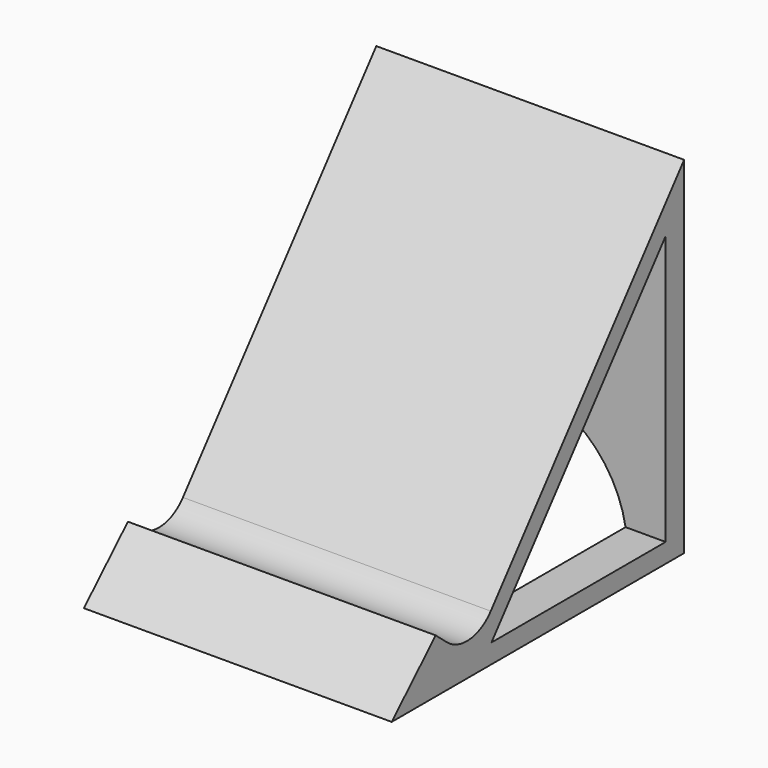
from build123d import *

# Parameters (mm, degrees)
F1_DEPTH = 101.6
F3_REACH = 205.8451899427


with BuildPart() as f1:
    # F0 (on Right) → F1 (new body)
    with BuildSketch(Plane.YZ):
        with BuildLine():
            Line((-36.1766421175, -23.2471508509), (-54.3283293044, -41.0144312356))
            Line((-54.3283293044, -41.0144312356), (58.7016706956, -41.0144312356))
            Line((58.7016706956, -41.0144312356), (58.7016706956, -34.6644312356))
            Line((58.7016706956, -34.6644312356), (-13.140378273, -34.6644312356))
            Line((-13.140378273, -34.6644312356), (58.7016706956, 54.2355687644))
            Line((58.7016706956, 54.2355687644), (66.3216706956, 54.2355687644))
            Line((66.3216706956, 54.2355687644), (66.3216706956, 73.2855687644))
            Line((66.3216706956, 73.2855687644), (-13.4575252541, -25.4361495295))
            ThreePointArc((-13.4575252541, -25.4361495295), (-22.1196896865, -30.0953879884), (-31.5109779006, -27.1721532474))
            Line((-31.5109779006, -27.1721532474), (-36.1766421175, -23.2471508509))
        make_face()
        Polygon((58.7016706956, -34.6644312356), (58.7016706956, -41.0144312356), (66.3216706956, -41.0144312356), (66.3216706956, 54.2355687644), (58.7016706956, 54.2355687644), align=None)
    extrude(amount=F1_DEPTH)

    f3_end = Plane(origin=(50.8, 22.7806462113, 9.7855687644), x_dir=(0, 0.6285393611, 0.7777777778), z_dir=(0, 0.7777777778, -0.6285393611))
    # F2 (on face) → F3 (cut, up to a plane its end follows)
    with BuildSketch(Plane(origin=(0, 66.3216706956, 0), x_dir=(-1, 0, 0), z_dir=(0, 1, 0))):
        with BuildLine():
            Line((-88.9, -41.0144312356), (-12.7, -41.0144312356))
            ThreePointArc((-12.7, -41.0144312356), (-50.8, -2.9144312356), (-88.9, -41.0144312356))
        make_face()
    f3_long = extrude(amount=-F3_REACH, mode=Mode.PRIVATE)
    add(split(f3_long, bisect_by=f3_end, keep=Keep.TOP, mode=Mode.PRIVATE), mode=Mode.SUBTRACT)


solid = f1.part
